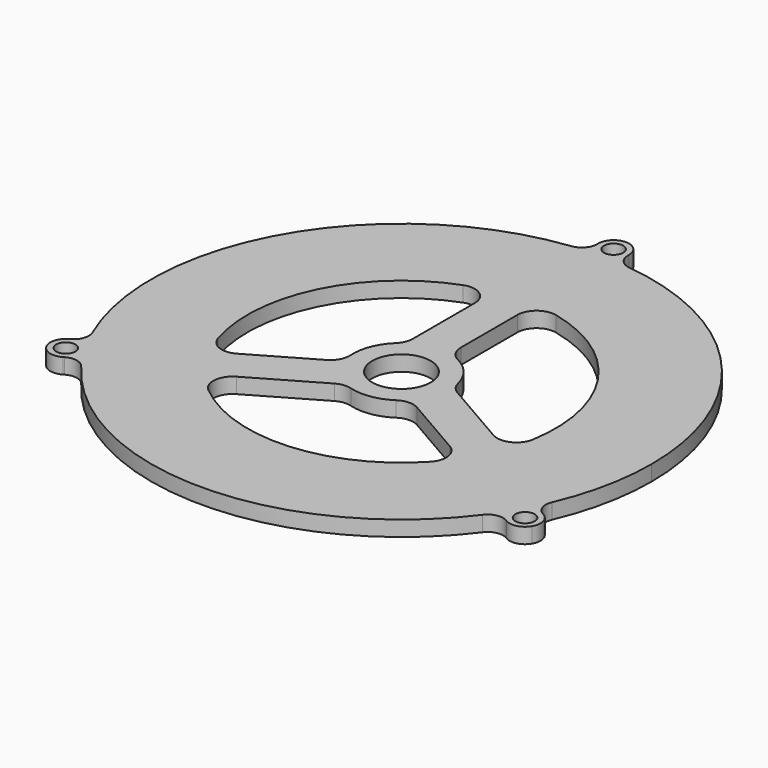
from build123d import *

# Parameters (mm, degrees)
F0_R     = 4.826
F0_R_2   = 1.5875
F1_DEPTH = 2.54
F2_R     = 2.53999


# Not quite as in the source:
# - a fillet or chamfer is up to 0.001 mm smaller than in the source, because OpenCascade refuses the exact size


with BuildPart() as f1:
    # F0 (on Top) → F1 (new body)
    with BuildSketch(Plane.XY):
        with BuildLine():
            ThreePointArc((36.9474511246, -18.3986814852), (40.1785494398, -9.4503857019), (41.275, 0))
            ThreePointArc((41.275, 0), (30.0704516511, 28.2735488133), (2.54, 41.1967720216))
            ThreePointArc((2.54, 41.1967720216), (0, 41.275), (-2.54, 41.1967720216))
            ThreePointArc((-2.54, 41.1967720216), (-35.7451985412, 20.6375), (-36.9474511246, -18.3986814852))
            ThreePointArc((-36.9474511246, -18.3986814852), (-35.7451985412, -20.6375), (-34.4074511246, -22.7980905364))
            ThreePointArc((-34.4074511246, -22.7980905364), (0, -41.275), (34.4074511246, -22.7980905364))
            ThreePointArc((34.4074511246, -22.7980905364), (35.7451985412, -20.6375), (36.9474511246, -18.3986814852))
        make_face()
        with BuildLine():
            ThreePointArc((-16.1831892187, -19.5771393904), (-17.3242054231, -16.864916263), (-15.7477905664, -14.3803663096))
            Line((-15.7477905664, -14.3803663096), (-4.6795539693, -7.9901169308))
            ThreePointArc((-4.6795539693, -7.9901169308), (-3.4772976031, -7.5882063232), (-2.2136295462, -7.6886829322))
            ThreePointArc((-2.2136295462, -7.6886829322), (1.2293114508, -7.9059973664), (4.4437139688, -6.6535259196))
            ThreePointArc((4.4437139688, -6.6535259196), (6.1035441451, -6.1205029783), (7.7945925279, -6.544183326))
            Line((7.7945925279, -6.544183326), (17.8798534353, -12.3669114257))
            ThreePointArc((17.8798534353, -12.3669114257), (19.431886995, -14.6433042701), (18.6198324975, -17.2760480945))
            ThreePointArc((18.6198324975, -17.2760480945), (1.6757275748, -25.3446628917), (-16.1831892187, -19.5771393904))
        make_face(mode=Mode.SUBTRACT)
        Circle(F0_R, mode=Mode.SUBTRACT)
        with BuildLine():
            ThreePointArc((-24.2714127756, -7.4872239098), (-22.786985702, 11.2211087963), (-8.8627054362, 23.8036226729))
            ThreePointArc((-8.8627054362, 23.8036226729), (-5.9433432049, 23.4356601283), (-4.5798672566, 20.8281698388))
            Line((-4.5798672566, 20.8281698388), (-4.5798672566, 8.0476710812))
            ThreePointArc((-4.5798672566, 8.0476710812), (-4.8329306435, 6.8055312224), (-5.5517799678, 5.7614008877))
            ThreePointArc((-5.5517799678, 5.7614008877), (-7.4614502869, 2.8883837376), (-7.9839794556, -0.5216062243))
            ThreePointArc((-7.9839794556, -0.5216062243), (-8.3522831357, -2.2255727936), (-9.5647252713, -3.4782234783))
            Line((-9.5647252713, -3.4782234783), (-19.6499861787, -9.3009515781))
            ThreePointArc((-19.6499861787, -9.3009515781), (-22.3974169907, -9.5068556461), (-24.2714127756, -7.4872239098))
        make_face(mode=Mode.SUBTRACT)
        with BuildLine():
            Line((1.7701327434, 10.0224068043), (1.7701327434, 21.6678630038))
            ThreePointArc((1.7701327434, 21.6678630038), (2.9655299957, 24.1501599162), (5.6515802781, 24.7632720043))
            ThreePointArc((5.6515802781, 24.7632720043), (21.1112581272, 14.1235540955), (25.0458946549, -4.2264832825))
            ThreePointArc((25.0458946549, -4.2264832825), (23.267548628, -6.5707438653), (20.327657823, -6.4478035292))
            Line((20.327657823, -6.4478035292), (9.259421226, -0.0575541504))
            ThreePointArc((9.259421226, -0.0575541504), (8.3102282466, 0.7826751008), (7.7654095141, 1.9272820445))
            ThreePointArc((7.7654095141, 1.9272820445), (6.2321388361, 5.0176136288), (3.5402654867, 7.175132144))
            ThreePointArc((3.5402654867, 7.175132144), (2.2487389906, 8.3460757719), (1.7701327434, 10.0224068043))
        make_face(mode=Mode.SUBTRACT)
        with BuildLine():
            ThreePointArc((-2.54, 41.1967720216), (0, 41.275), (2.54, 41.1967720216))
            Line((2.54, 41.1967720216), (2.54, 46.2767720216))
            Line((2.54, 46.2767720216), (-2.54, 46.2767720216))
            Line((-2.54, 46.2767720216), (-2.54, 41.1967720216))
        make_face()
        with Locations((0, 43.7367720216)):
            Circle(F0_R_2, mode=Mode.SUBTRACT)
        with BuildLine():
            ThreePointArc((-34.4074511246, -22.7980905364), (-35.7451985412, -20.6375), (-36.9474511246, -18.3986814852))
            Line((-36.9474511246, -18.3986814852), (-41.3468601758, -20.9386814852))
            Line((-41.3468601758, -20.9386814852), (-38.8068601758, -25.3380905364))
            Line((-38.8068601758, -25.3380905364), (-34.4074511246, -22.7980905364))
        make_face()
        with Locations((-37.8771556502, -21.8683860108)):
            Circle(F0_R_2, mode=Mode.SUBTRACT)
        with BuildLine():
            Line((41.3468601758, -20.9386814852), (36.9474511246, -18.3986814852))
            ThreePointArc((36.9474511246, -18.3986814852), (35.7451985412, -20.6375), (34.4074511246, -22.7980905364))
            Line((34.4074511246, -22.7980905364), (38.8068601758, -25.3380905364))
            Line((38.8068601758, -25.3380905364), (41.3468601758, -20.9386814852))
        make_face()
        with Locations((37.8771556502, -21.8683860108)):
            Circle(F0_R_2, mode=Mode.SUBTRACT)
    extrude(amount=F1_DEPTH)

    # F2 (radius 2.54 in the source; OpenCascade refuses exactly that, so slightly less here)
    f2_edges = [f1.edges().sort_by_distance(p)[0] for p in [
        (-34.407451, -22.798091, 1.27),
        (-38.80686, -25.338091, 1.27),
        (-41.34686, -20.938681, 1.27),
        (-36.947451, -18.398681, 1.27),
        (34.407451, -22.798091, 1.27),
        (38.80686, -25.338091, 1.27),
        (41.34686, -20.938681, 1.27),
        (36.947451, -18.398681, 1.27),
        (2.54, 41.196772, 1.27),
        (2.54, 46.276772, 1.27),
        (-2.54, 41.196772, 1.27),
        (-2.54, 46.276772, 1.27),
    ]]
    fillet(f2_edges, radius=F2_R)


solid = f1.part
